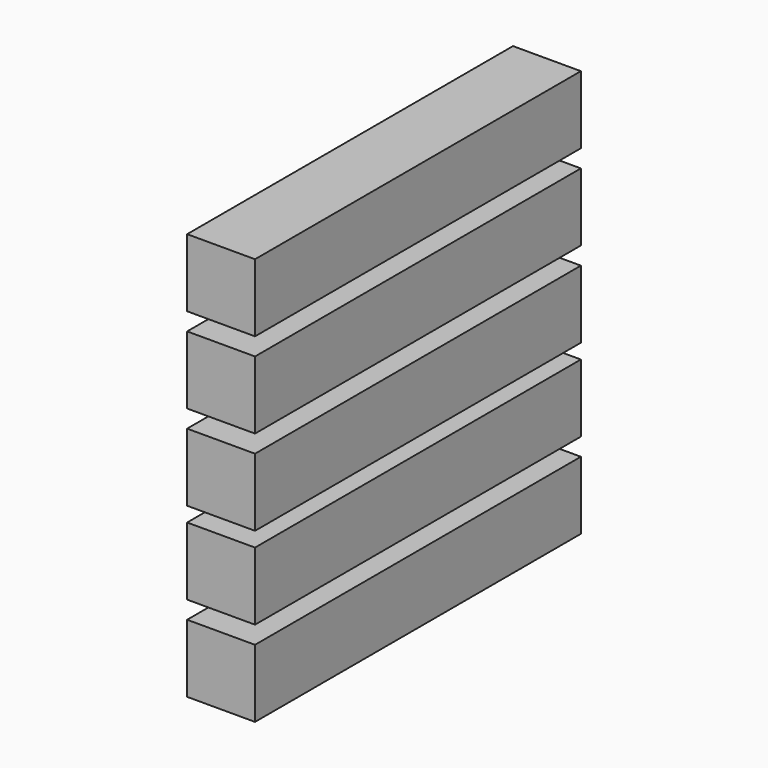
from build123d import *

# Parameters (mm, degrees)
F1_DEPTH = 5
F0_W     = 30
F0_H     = 5.0000004371
F0_H_2   = 5


# Not quite as in the source:
# - ends of sketch curves that miss each other by under 0.0002 mm in the source are joined


with BuildPart() as f1:
    # F0 (on Right) → F1 (new body)
    with BuildSketch(Plane.YZ):
        Polygon((0, -25.0000003725), (0, -30), (12, -30), (12.39, -30), (12.4011761725, -30), (17.61, -30), (30, -30), (30, -25.0000003725), align=None)
    extrude(amount=F1_DEPTH)


with BuildPart() as f1b:
    # F0 (on Right) → F1, piece 2 (new body)
    with BuildSketch(Plane.YZ):
        with Locations((15, -21.195660154)):
            Rectangle(F0_W, F0_H)
    extrude(amount=F1_DEPTH)


with BuildPart() as f1c:
    # F0 (on Right) → F1, piece 3 (new body)
    with BuildSketch(Plane.YZ):
        with Locations((15, -15.10868)):
            Rectangle(F0_W, F0_H_2)
    extrude(amount=F1_DEPTH)


with BuildPart() as f1d:
    # F0 (on Right) → F1, piece 4 (new body)
    with BuildSketch(Plane.YZ):
        with Locations((15, -8.80434)):
            Rectangle(F0_W, F0_H_2)
    extrude(amount=F1_DEPTH)


with BuildPart() as f1e:
    # F0 (on Right) → F1, piece 5 (new body)
    with BuildSketch(Plane.YZ):
        Polygon((6.5217, 0), (0, 0), (0, -5), (30, -5), (30, 0), (23.4783, 0), align=None)
    extrude(amount=F1_DEPTH)


solid = Compound([f1.part, f1b.part, f1c.part, f1d.part, f1e.part])
